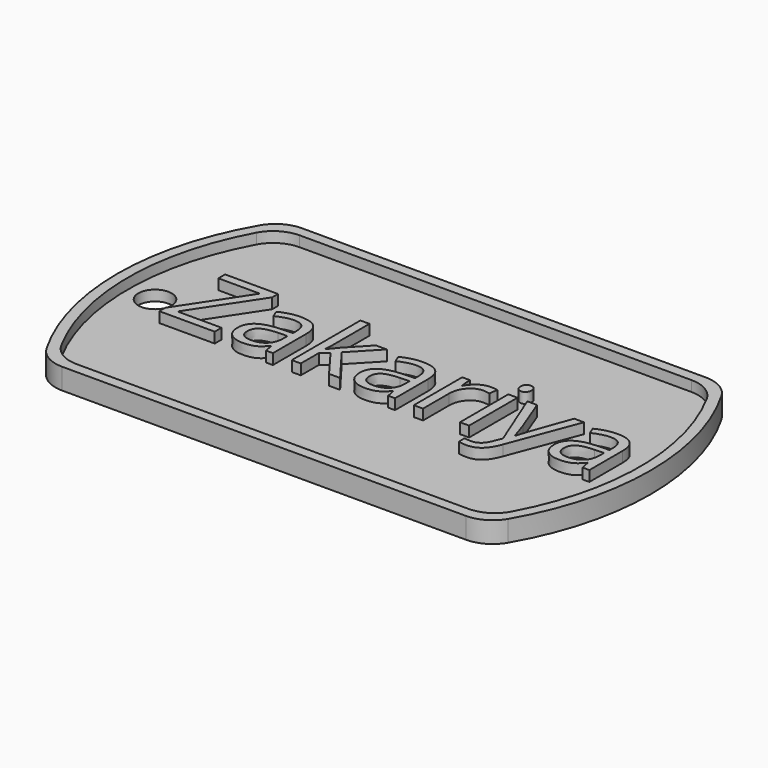
from build123d import *

# Parameters (mm, degrees)
F1_DEPTH     = 1
F3_DEPTH     = 1
F4_R         = 1.5875
F5_DEPTH     = 1
F6_TEXT_SIZE = 10.7627142117
F7_DEPTH     = 1


# Not quite as in the source:
# - Text() gives the source's letters only with a copy of the font that has no kerning and outlines rounded to 1/6400 em; it was checked with that copy


with BuildPart() as f1:
    # F0 (on Top) → F1 (new body)
    with BuildSketch(Plane.XY):
        with BuildLine():
            ThreePointArc((-19.2474145991, 14.2875), (-20.8349145991, 13.862130657), (-21.9970452561, 12.7))
            ThreePointArc((-21.9970452561, 12.7), (-25.4, 0), (-21.9970452561, -12.7))
            ThreePointArc((-21.9970452561, -12.7), (-20.8349145991, -13.862130657), (-19.2474145991, -14.2875))
            Line((-19.2474145991, -14.2875), (19.2474145991, -14.2875))
            ThreePointArc((19.2474145991, -14.2875), (20.8349145991, -13.862130657), (21.9970452561, -12.7))
            ThreePointArc((21.9970452561, -12.7), (25.4, 0), (21.9970452561, 12.7))
            ThreePointArc((21.9970452561, 12.7), (20.8349145991, 13.862130657), (19.2474145991, 14.2875))
            Line((19.2474145991, 14.2875), (-19.2474145991, 14.2875))
        make_face()
    extrude(amount=F1_DEPTH)

    # F2 (on face) → F3 (join)
    with BuildSketch(Plane.XY.offset(1)):
        with BuildLine():
            Line((19.2474145991, 14.2875), (-19.2474145991, 14.2875))
            ThreePointArc((-19.2474145991, 14.2875), (-20.8349145991, 13.862130657), (-21.9970452561, 12.7))
            ThreePointArc((-21.9970452561, 12.7), (-25.4, 0), (-21.9970452561, -12.7))
            ThreePointArc((-21.9970452561, -12.7), (-20.8349145991, -13.862130657), (-19.2474145991, -14.2875))
            Line((-19.2474145991, -14.2875), (19.2474145991, -14.2875))
            ThreePointArc((19.2474145991, -14.2875), (20.8349145991, -13.862130657), (21.9970452561, -12.7))
            ThreePointArc((21.9970452561, -12.7), (25.4, 0), (21.9970452561, 12.7))
            ThreePointArc((21.9970452561, 12.7), (20.8349145991, 13.862130657), (19.2474145991, 14.2875))
        make_face()
        with BuildLine():
            ThreePointArc((-21.4526124879, 11.6252061249), (-20.2856017842, 12.8404540819), (-18.6611352482, 13.2875))
            Line((-18.6611352482, 13.2875), (18.6611352482, 13.2875))
            ThreePointArc((18.6611352482, 13.2875), (20.2856017842, 12.8404540819), (21.4526124879, 11.6252061249))
            ThreePointArc((21.4526124879, 11.6252061249), (24.4, 0), (21.4526124879, -11.6252061249))
            ThreePointArc((21.4526124879, -11.6252061249), (20.2856017842, -12.8404540819), (18.6611352482, -13.2875))
            Line((18.6611352482, -13.2875), (-18.6611352482, -13.2875))
            ThreePointArc((-18.6611352482, -13.2875), (-20.2856017842, -12.8404540819), (-21.4526124879, -11.6252061249))
            ThreePointArc((-21.4526124879, -11.6252061249), (-24.4, 0), (-21.4526124879, 11.6252061249))
        make_face(mode=Mode.SUBTRACT)
    extrude(amount=F3_DEPTH)

    # F4 (on face) → F5 (cut)
    with BuildSketch(Plane.XY.offset(1)):
        with Locations((-21.821282804, 0)):
            Circle(F4_R)
    extrude(amount=-F5_DEPTH, mode=Mode.SUBTRACT)

    # F6 (on face) → F7 (join)
    with BuildSketch(Plane.XY.offset(1)):
        with Locations((-19.6190122515, -2.7802931145)):
            Text('Zakariya', F6_TEXT_SIZE, font='Open Sans', text_align=(TextAlign.LEFT, TextAlign.BOTTOM))
    extrude(amount=F7_DEPTH)


solid = f1.part
